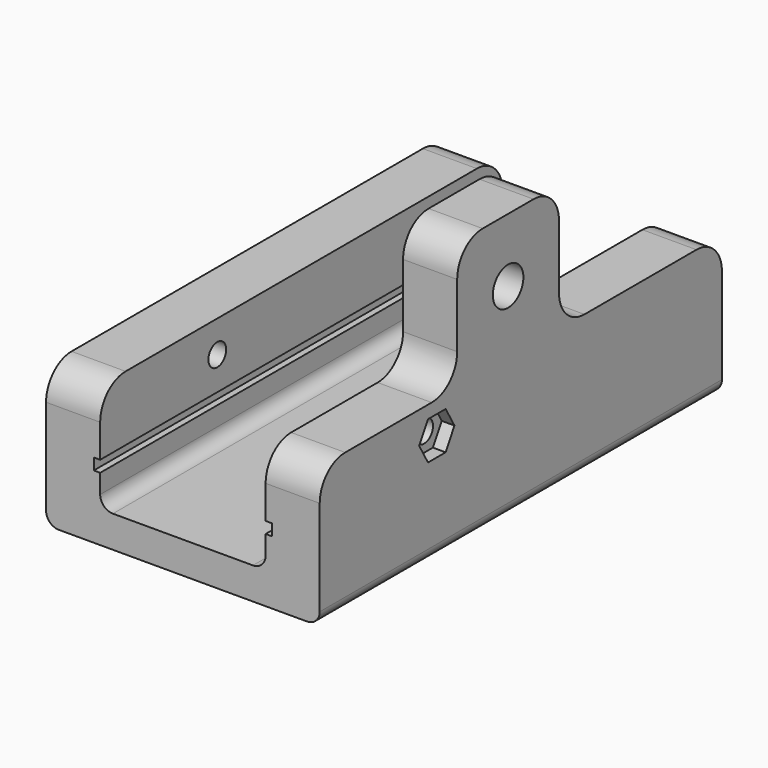
from build123d import *

# Parameters (mm, degrees)
F0_W      = 43
F0_H      = 79
F0_W_2    = 28
F0_H_2    = 64
F1_DEPTH  = 22
F2_W      = 26
F2_H      = 10.2
F2_H_2    = 1.8
F2_H_3    = 5
F2_W_2    = 1
F3_DEPTH  = 100
F4_R      = 1.75
F5_DEPTH  = 100
F4_R_2    = 3
F6_DEPTH  = 2
F7_R      = 1.75
F8_DEPTH  = 2
F9_W      = 8.5
F9_H      = 20
F10_DEPTH = 20
F11_R     = 3
F12_DEPTH = 25
F13_SIZE  = 2
F14_R     = 5
F15_R     = 2


# Not quite as in the source:
# - a feature names something its author has since deleted; it is built from what else it names


with BuildPart() as f1:
    # F0 (on Top) → F1 (new body)
    with BuildSketch(Plane.XY):
        Rectangle(F0_W, F0_H)
        Rectangle(F0_W_2, F0_H_2, mode=Mode.SUBTRACT)
        Rectangle(F0_W_2, F0_H_2)
    extrude(amount=F1_DEPTH)

    # F2 (on face) → F3 (cut)
    with BuildSketch(Plane.XZ.offset(39.5)):
        with Locations((0, 16.9)):
            Rectangle(F2_W, F2_H)
        with Locations((0, 10.9)):
            Rectangle(F2_W, F2_H_2)
        with Locations((0, 7.5)):
            Rectangle(F2_W, F2_H_3)
        with Locations((-13.5, 10.9)):
            Rectangle(F2_W_2, F2_H_2)
        with Locations((13.5, 10.9)):
            Rectangle(F2_W_2, F2_H_2)
    extrude(amount=-F3_DEPTH, mode=Mode.SUBTRACT)

    # F4 (on face) → F5 (cut)
    with BuildSketch(Plane(origin=(-21.5, 0, 0), x_dir=(0, -1, 0), z_dir=(-1, 0, 0))):
        with Locations((16.5, 17)):
            Circle(F4_R)
    extrude(amount=-F5_DEPTH, mode=Mode.SUBTRACT)

    # F4 (on face) → F6 (cut)
    with BuildSketch(Plane(origin=(-21.5, 0, 0), x_dir=(0, -1, 0), z_dir=(-1, 0, 0))):
        with Locations((16.5, 17)):
            Circle(F4_R_2)
        with Locations((16.5, 17)):
            Circle(F4_R, mode=Mode.SUBTRACT)
    extrude(amount=-F6_DEPTH, mode=Mode.SUBTRACT)

    # F7 (on face) → F8 (cut)
    with BuildSketch(Plane.YZ.offset(21.5)):
        Polygon((-18.2320508076, 14), (-14.7679491924, 14), (-13.0358983849, 17), (-14.7679491924, 20), (-18.2320508076, 20), (-19.9641016151, 17), align=None)
        with Locations((-16.5, 17)):
            Circle(F7_R, mode=Mode.SUBTRACT)
    extrude(amount=-F8_DEPTH, mode=Mode.SUBTRACT)

    # F9 (on face) → F10 (join)
    with BuildSketch(Plane.XY.offset(22)):
        with Locations((17.25, -2.5)):
            Rectangle(F9_W, F9_H)
    extrude(amount=F10_DEPTH)

    # F11 (on face) → F12 (cut)
    with BuildSketch(Plane.YZ.offset(21.5)):
        with Locations((-2.5, 32)):
            Circle(F11_R)
    extrude(amount=-F12_DEPTH, mode=Mode.SUBTRACT)

    # F13
    f13_edges = [f1.edges().sort_by_distance(p)[0] for p in [
        (13, -5.5, 32),
    ]]
    chamfer(f13_edges, length=F13_SIZE)

    # F14
    f14_edges = [f1.edges().sort_by_distance(p)[0] for p in [
        (17.25, 7.5, 42),
        (17.25, -12.5, 42),
        (17.25, -12.5, 22),
        (17.25, 7.5, 22),
        (17.25, 39.5, 22),
        (17.25, -39.5, 22),
        (-17.25, -39.5, 22),
        (-17.25, 39.5, 22),
    ]]
    fillet(f14_edges, radius=F14_R)

    # F15
    f15_edges = [f1.edges().sort_by_distance(p)[0] for p in [
        (13, 0, 5),
        (-13, 0, 5),
        (21.5, 0, 0),
        (-21.5, 0, 0),
    ]]
    fillet(f15_edges, radius=F15_R)


solid = f1.part
